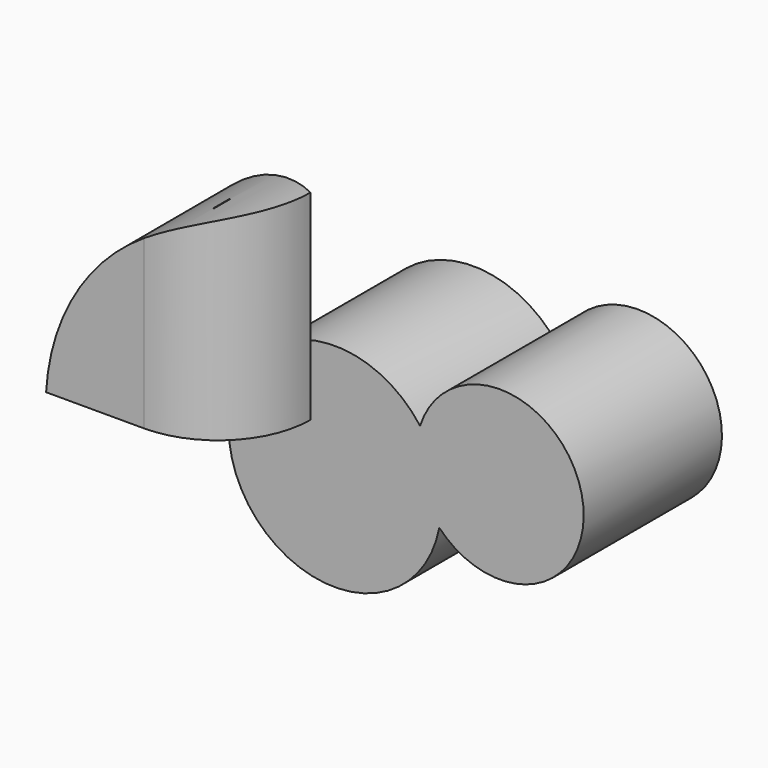
from build123d import *

# Parameters (mm, degrees)
F0_W        = 44.3030558527
F0_H        = 33.7232230231
F0_W_2      = 0.2780174837
F0_H_2      = 4.7262893058
F1_DEPTH    = 46.482
F2_T1_DEPTH = 280.6193273788
F3_R        = 21.4623585695
F4_T1_DEPTH = 270.9255150881
F6_DEPTH    = 40.132


# Not quite as in the source:
# - a fillet or chamfer that OpenCascade refuses, or shapes differently, is made with other operations: its cross-section is extruded or revolved along the edge and cut away or added


with BuildPart() as f1:
    # F0 (on Top) → F1 (new body)
    with BuildSketch(Plane.XY):
        with Locations((0.330619514, -6.2817768194)):
            Rectangle(F0_W, F0_H)
        with Locations((8.0964784138, -9.5091590192)):
            Rectangle(F0_W_2, F0_H_2, mode=Mode.SUBTRACT)
    extrude(amount=F1_DEPTH)

    # F2: fillet of radius 49.6700298323 on 1 edges, made by hand

    # F2_s2 → F2_t1 (cut)
    with BuildSketch(Plane.XZ.offset(-134.02788687)):
        with BuildLine():
            ThreePointArc((-21.8209084123, -2.8972208711), (-9.1217429277, 30.2730527625), (22.4821474403, 46.482))
            Line((22.4821474403, 46.482), (-21.8209084123, 46.482))
            Line((-21.8209084123, 46.482), (-21.8209084123, -2.8972208711))
        make_face()
    extrude(amount=F2_T1_DEPTH, mode=Mode.SUBTRACT)

    # F3
    f3_edges = [f1.edges().sort_by_distance(p)[0] for p in [
        (22.482147, -23.143388, 23.241),
    ]]
    fillet(f3_edges, radius=F3_R)

    # F4: fillet of radius 88.3022752574 on 2 edges, made by hand

    # F4_s2 → F4_t1 (cut)
    with BuildSketch(Plane.XY.offset(-112.221757544)):
        with BuildLine():
            ThreePointArc((22.4821474403, -1.6810297614), (0.8599678832, 7.4594865185), (-22.4065555773, 10.5798346922))
            Line((-22.4065555773, 10.5798346922), (22.4821474403, 10.5798346922))
            Line((22.4821474403, 10.5798346922), (22.4821474403, -1.6810297614))
        make_face()
    extrude(amount=F4_T1_DEPTH, mode=Mode.SUBTRACT)

    # F5 (on Front) → F6 (join)
    with BuildSketch(Plane.XZ):
        with BuildLine():
            ThreePointArc((51.0496692561, -13.4370785738), (51.3779423625, -11.1330198173), (51.4876921444, -8.808282204))
            ThreePointArc((51.4876921444, -8.808282204), (50.2324406688, -1.038184698), (46.594391977, 5.9414050633))
            ThreePointArc((46.594391977, 5.9414050633), (46.1598632778, -4.3598915413), (51.0496692561, -13.4370785738))
        make_face()
        with BuildLine():
            ThreePointArc((46.594391977, 5.9414050633), (50.2324406688, -1.038184698), (51.4876921444, -8.808282204))
            ThreePointArc((51.4876921444, -8.808282204), (51.3779423625, -11.1330198173), (51.0496692561, -13.4370785738))
            ThreePointArc((51.0496692561, -13.4370785738), (72.3613537789, -18.0621042721), (84.58179359, 0))
            ThreePointArc((84.58179359, 0), (68.1302794475, 19.2246129703), (46.594391977, 5.9414050633))
        make_face()
        with BuildLine():
            ThreePointArc((51.0496692561, -13.4370785738), (46.1598632778, -4.3598915413), (46.594391977, 5.9414050633))
            ThreePointArc((46.594391977, 5.9414050633), (2.7623791307, -14.3373401751), (51.0496692561, -13.4370785738))
        make_face()
    extrude(amount=-F6_DEPTH)


solid = f1.part
